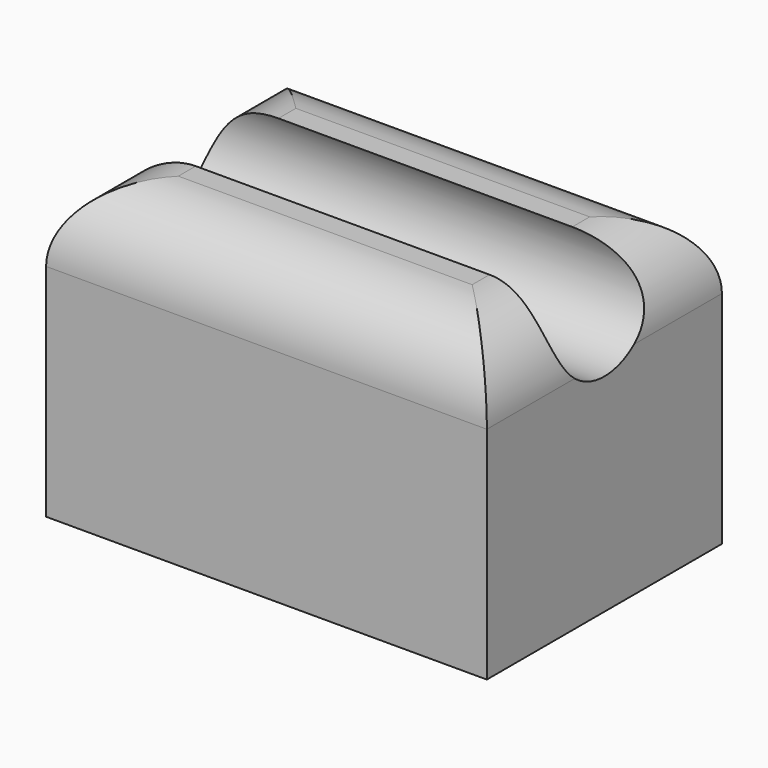
from build123d import *

# Parameters (mm, degrees)
F0_W     = 20
F0_H     = 20
F1_DEPTH = 30
F3_D     = 8
F3_DEPTH = 50
F3_TIP   = 2.4034424761
F4_R     = 5
F5_W     = 20
F5_H     = 13
F6_DEPTH = 0.5


# Not quite as in the source:
# - a feature names something its author has since deleted; it is built from what else it names


with BuildPart() as f1:
    # F0 (on Right) → F1 (new body)
    with BuildSketch(Plane.YZ):
        with Locations((-10, 10)):
            Rectangle(F0_W, F0_H)
    extrude(amount=F1_DEPTH)

    # F3
    with Locations(Plane.YZ.offset(30)):
        with Locations((-10, 18.097827211)):
            Hole(F3_D / 2, depth=F3_DEPTH)
            with Locations((0, 0, -(F3_DEPTH + F3_TIP / 2))):  # 118° drill point
                Cone(0, F3_D / 2, F3_TIP, mode=Mode.SUBTRACT)

    # F4
    f4_edges = [f1.edges().sort_by_distance(p)[0] for p in [
        (30, -3.240615, 20),
        (30, -16.759385, 20),
        (15, -20, 20),
        (15, 0, 20),
        (0, -16.759385, 20),
        (0, -3.240615, 20),
    ]]
    fillet(f4_edges, radius=F4_R)

    # F5 (on face) → F6 (cut)
    with BuildSketch(Plane(origin=(0, 0, 0), x_dir=(1, 0, 0), z_dir=(0, 0, -1))):
        with Locations((15, 9.8333333333)):
            Rectangle(F5_W, F5_H)
    extrude(amount=-F6_DEPTH, mode=Mode.SUBTRACT)


solid = f1.part
